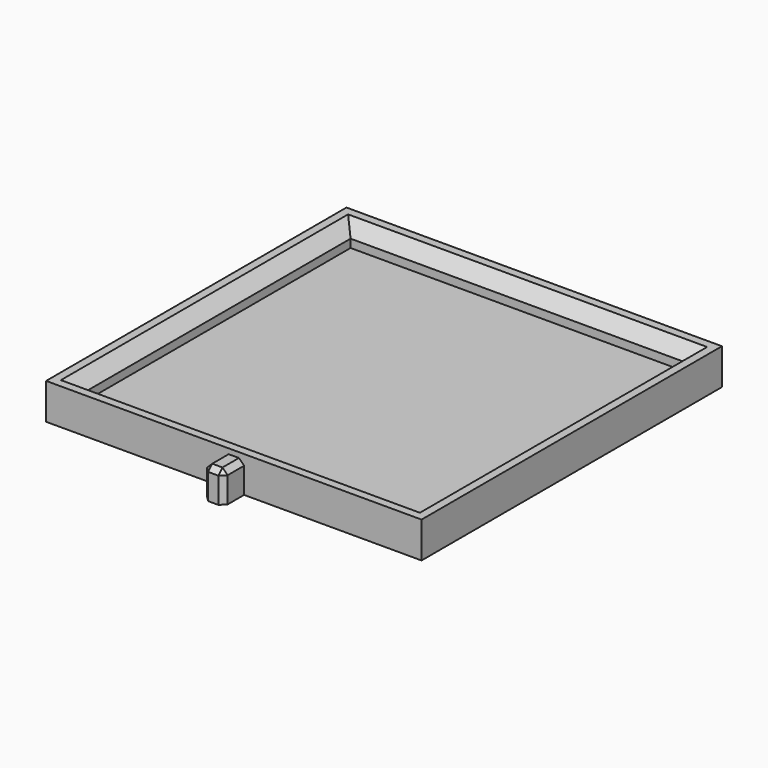
from build123d import *

# Parameters (mm, degrees)
F1_DEPTH = 41.275
F2_W     = 82.55
F2_H     = 5.08
F3_DEPTH = 5.08
F4_W     = 92.71
F4_H     = 8.89
F5_DEPTH = 5.08
F6_W     = 5.0743944012
F6_H     = 7.62
F7_DEPTH = 6.35
F8_SIZE  = 1.27
F9_SIZE  = 3.048


with BuildPart() as f1:
    # F0 (on Front) → F1 (new body, symmetric)
    with BuildSketch(Plane.XZ):
        Polygon((-41.275, -3.81), (-41.275, 0), (-41.275, 5.08), (-46.355, 5.08), (-46.355, -3.81), align=None)
        Polygon((41.275, 0), (0, 0), (-41.275, 0), (-41.275, -3.81), (41.275, -3.81), align=None)
        Polygon((41.275, 5.08), (41.275, 0), (41.275, -3.81), (46.355, -3.81), (46.355, 5.08), align=None)
    extrude(amount=F1_DEPTH, both=True)

    # F2 (on face) → F3 (join)
    with BuildSketch(Plane.XZ.offset(41.275)):
        Polygon((-46.355, 5.08), (-46.355, -3.81), (46.355, -3.81), (46.355, 5.08), (41.275, 5.08), (41.275, 0), (-41.275, 0), (-41.275, 5.08), align=None)
        with Locations((0, 2.54)):
            Rectangle(F2_W, F2_H)
    extrude(amount=F3_DEPTH)

    # F4 (on face) → F5 (join)
    with BuildSketch(Plane(origin=(0, 41.275, 0), x_dir=(-1, 0, 0), z_dir=(0, 1, 0))):
        with Locations((0, 0.635)):
            Rectangle(F4_W, F4_H)
    extrude(amount=F5_DEPTH)

    # F6 (on face) → F7 (join)
    with BuildSketch(Plane.XZ.offset(46.355)):
        Rectangle(F6_W, F6_H)
    extrude(amount=F7_DEPTH)

    # F8
    f8_edges = [f1.edges().sort_by_distance(p)[0] for p in [
        (-2.537197, -49.53, 3.81),
        (2.537197, -49.53, 3.81),
        (0, -52.705, 3.81),
        (2.537197, -52.705, 0),
        (-2.537197, -52.705, 0),
    ]]
    chamfer(f8_edges, length=F8_SIZE)

    # F9
    f9_edges = [f1.edges().sort_by_distance(p)[0] for p in [
        (-41.275, 0, 5.08),
        (0, 41.275, 5.08),
        (0, -41.275, 5.08),
        (41.275, 0, 5.08),
    ]]
    chamfer(f9_edges, length=F9_SIZE)


solid = f1.part
